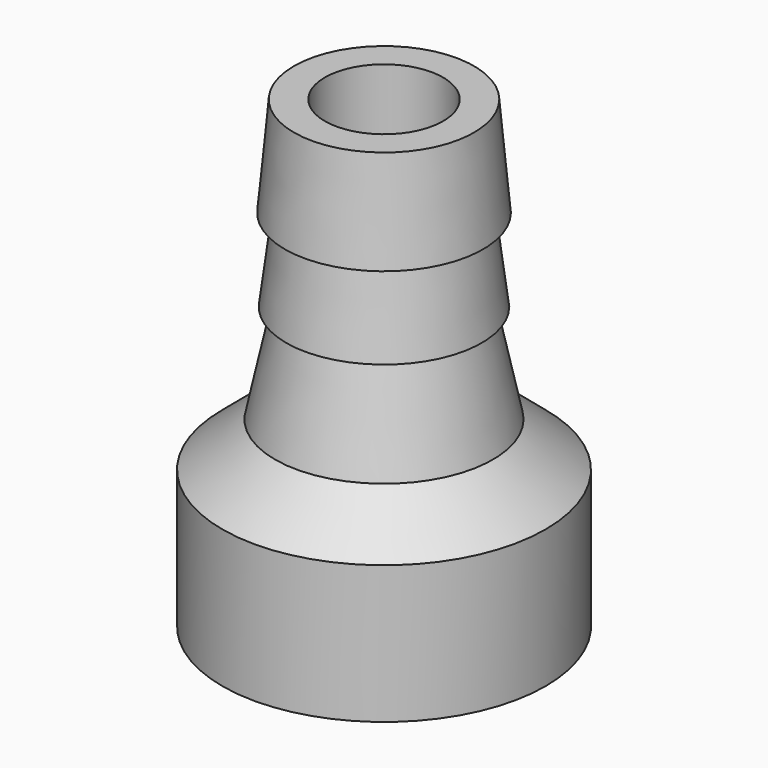
from build123d import *

# Parameters (mm, degrees)
F2_SIZE = 0.99999


# Not quite as in the source:
# - a fillet or chamfer is up to 0.001 mm smaller than in the source, because OpenCascade refuses the exact size


with BuildPart() as f1:
    # F0 (on Front) → F1 (revolve)
    with BuildSketch(Plane.XZ):
        with BuildLine():
            Line((-8.2, -1.5365384456), (-6.2, -1.5365384456))
            Line((-6.2, -1.5365384456), (-6.2, -0.5365384456))
            ThreePointArc((-6.2, -0.5365384456), (-5.7, -0.0365384456), (-6.2, 0.4634615544))
            Line((-6.2, 0.4634615544), (-6.2, 1.4634615544))
            ThreePointArc((-6.2, 1.4634615544), (-5.7, 1.9634615544), (-6.2, 2.4634615544))
            Line((-6.2, 2.4634615544), (-6.2, 4.5634615544))
            Line((-6.2, 4.5634615544), (-3, 7.2563952203))
            Line((-3, 7.2563952203), (-3, 22))
            Line((-3, 22), (-4.566712814, 22))
            Line((-4.566712814, 22), (-5.0262918188, 16.9351019463))
            Line((-5.0262918188, 16.9351019463), (-4.4613682133, 16.7352703944))
            Line((-4.4613682133, 16.7352703944), (-4.9613682133, 12.7352703944))
            Line((-4.9613682133, 12.7352703944), (-4.4619254344, 12.7116714393))
            Line((-4.4619254344, 12.7116714393), (-5.5284631097, 7.7116714393))
            Line((-5.5284631097, 7.7116714393), (-8.2, 5.4634615544))
            Line((-8.2, 5.4634615544), (-8.2, -1.5365384456))
        make_face()
    revolve(axis=Axis((0, 0, 11), (0, 0, -1)))

    # F2 (size 1 in the source; OpenCascade refuses exactly that, so slightly less here)
    f2_edges = [f1.edges().sort_by_distance(p)[0] for p in [
        (6.2, 0, -1.536538),
    ]]
    chamfer(f2_edges, length=F2_SIZE)


solid = f1.part
